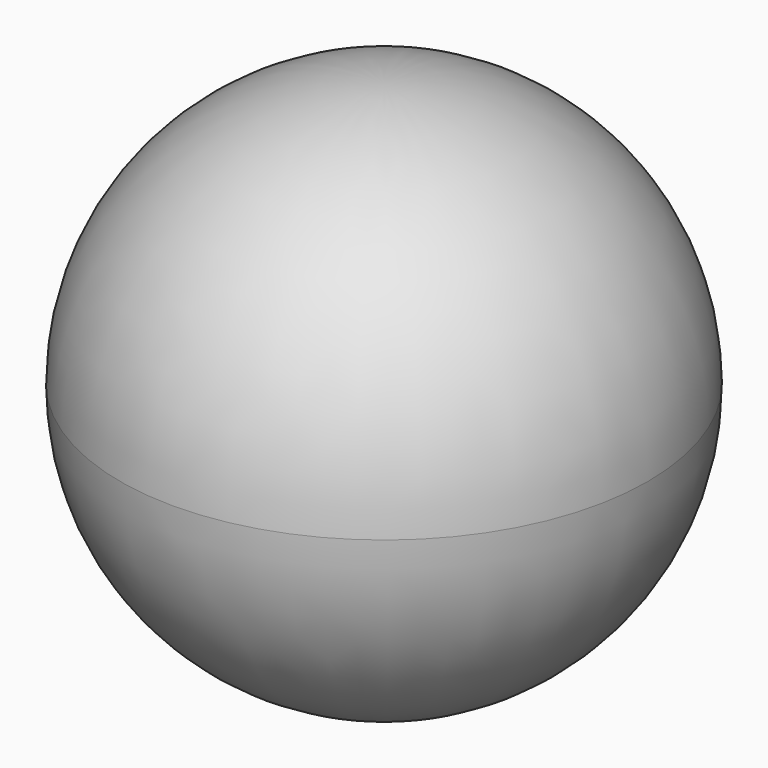
from build123d import *

# Parameters (mm, degrees)
F0_R     = 76.2
F1_DEPTH = 76.2
F2_DEPTH = 76.2
F3_R     = 76.19999


# Not quite as in the source:
# - a fillet or chamfer is up to 0.001 mm smaller than in the source, because OpenCascade refuses the exact size


with BuildPart() as f1:
    # F0 (on Top) → F1 (new body)
    with BuildSketch(Plane.XY):
        Circle(F0_R)
    extrude(amount=F1_DEPTH)

    # F2 (add): a face of the model
    f2_faces = [f1.faces().sort_by_distance(p)[0] for p in [
        (0, 0, 0),
    ]]
    extrude(f2_faces, amount=F2_DEPTH)

    # F3 (radius 76.2 in the source; OpenCascade refuses exactly that, so slightly less here)
    f3_edges = [f1.edges().sort_by_distance(p)[0] for p in [
        (-76.2, 0, -76.2),
        (-76.2, 0, 76.2),
    ]]
    fillet(f3_edges, radius=F3_R)


solid = f1.part
